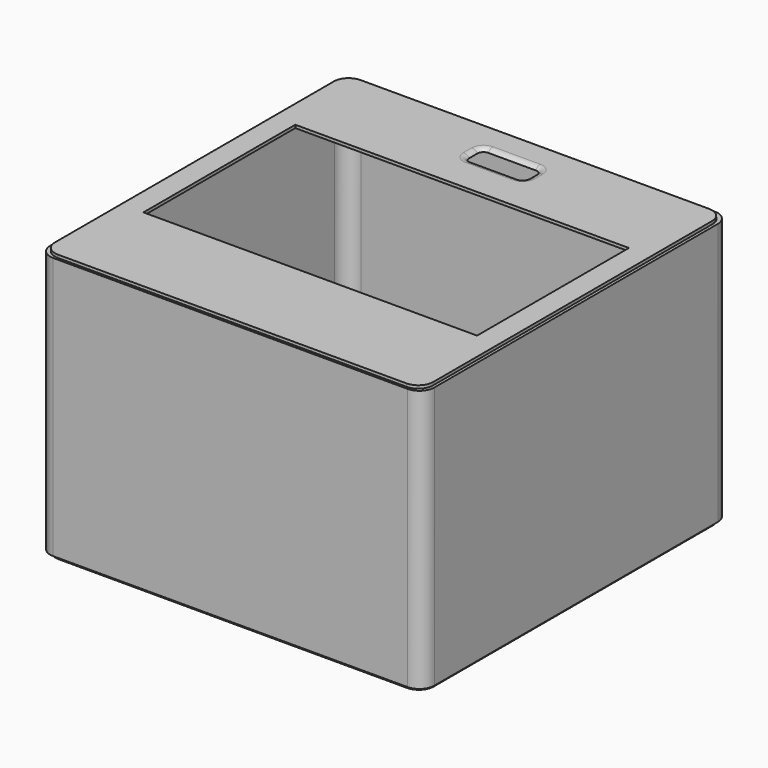
from build123d import *

# Parameters (mm, degrees)
F0_W         = 225
F0_H         = 128
F1_DEPTH     = 2
F2_T1_DEPTH  = 32
F2_T3_DEPTH  = 7
F2_T6_ANGLE  = 90
F2_T8_ANGLE  = 90
F2_T10_ANGLE = 90
F2_T12_ANGLE = 90
F4_DEPTH     = 177
F6_DEPTH     = 2


# Not quite as in the source:
# - a fillet or chamfer that OpenCascade refuses, or shapes differently, is made with other operations: its cross-section is extruded or revolved along the edge and cut away or added


with BuildPart() as f1:
    # F0 (on Top) → F1 (new body)
    with BuildSketch(Plane.XY):
        with BuildLine():
            Line((-120, -130), (115, -130))
            ThreePointArc((115, -130), (122.0710678119, -127.0710678119), (125, -120))
            Line((125, -120), (125, 115))
            ThreePointArc((125, 115), (122.0710678119, 122.0710678119), (115, 125))
            Line((115, 125), (-120, 125))
            ThreePointArc((-120, 125), (-127.0710678119, 122.0710678119), (-130, 115))
            Line((-130, 115), (-130, -120))
            ThreePointArc((-130, -120), (-127.0710678119, -127.0710678119), (-120, -130))
        make_face()
        with Locations((-2.5000095367, -0.2505254149)):
            Rectangle(F0_W, F0_H, mode=Mode.SUBTRACT)
        with BuildLine():
            Line((-18.0000054687, 105.1618295312), (13.9999945313, 105.1618295312))
            ThreePointArc((13.9999945313, 105.1618295312), (16.828421656, 103.9902566559), (17.9999945313, 101.1618295312))
            Line((17.9999945313, 101.1618295312), (17.9999945313, 94.1618295312))
            ThreePointArc((17.9999945313, 94.1618295312), (16.828421656, 91.3334024064), (13.9999945313, 90.1618295312))
            Line((13.9999945313, 90.1618295312), (-18.0000054687, 90.1618295312))
            ThreePointArc((-18.0000054687, 90.1618295312), (-20.8284325935, 91.3334024064), (-22.0000054687, 94.1618295312))
            Line((-22.0000054687, 94.1618295312), (-22.0000054687, 101.1618295312))
            ThreePointArc((-22.0000054687, 101.1618295312), (-20.8284325935, 103.9902566559), (-18.0000054687, 105.1618295312))
        make_face(mode=Mode.SUBTRACT)
    extrude(amount=F1_DEPTH)

    # F2: fillet of radius 5 on 1 edges, made by hand

    # F2_s2 → F2_t1 (cut)
    with BuildSketch(Plane.YZ.offset(-18.0000054687)):
        with BuildLine():
            ThreePointArc((90.1618295312, 0), (88.3978975087, 1.472135955), (86.1618295312, 2))
            Line((86.1618295312, 2), (90.1618295312, 2))
            Line((90.1618295312, 2), (90.1618295312, 0))
        make_face()
        with BuildLine():
            ThreePointArc((105.1618295312, 0), (106.9257615537, 1.472135955), (109.1618295312, 2))
            Line((109.1618295312, 2), (105.1618295312, 2))
            Line((105.1618295312, 2), (105.1618295312, 0))
        make_face()
    extrude(amount=F2_T1_DEPTH, mode=Mode.SUBTRACT)

    # F2_s4 → F2_t3 (cut)
    with BuildSketch(Plane.XZ.offset(-101.1618295312)):
        with BuildLine():
            ThreePointArc((-22.0000054687, 0), (-23.7639374912, 1.472135955), (-26.0000054687, 2))
            Line((-26.0000054687, 2), (-22.0000054687, 2))
            Line((-22.0000054687, 2), (-22.0000054687, 0))
        make_face()
        with BuildLine():
            ThreePointArc((17.9999945313, 0), (19.7639265538, 1.472135955), (21.9999945313, 2))
            Line((21.9999945313, 2), (17.9999945313, 2))
            Line((17.9999945313, 2), (17.9999945313, 0))
        make_face()
    extrude(amount=F2_T3_DEPTH, mode=Mode.SUBTRACT)

    # F2_s5 → F2_t6 (revolve, cut)
    with BuildSketch(Plane.XZ.offset(-94.1618295312)):
        with BuildLine():
            ThreePointArc((17.9999945313, 0), (19.7639265538, 1.472135955), (21.9999945313, 2))
            Line((21.9999945313, 2), (17.9999945313, 2))
            Line((17.9999945313, 2), (17.9999945313, 0))
        make_face()
    revolve(axis=Axis((13.9999945313, 94.1618295312, 2), (0, 0, -1)), revolution_arc=F2_T6_ANGLE, mode=Mode.SUBTRACT)

    # F2_s7 → F2_t8 (revolve, cut)
    with BuildSketch(Plane.YZ.offset(-18.0000054687)):
        with BuildLine():
            ThreePointArc((90.1618295312, 0), (88.3978975087, 1.472135955), (86.1618295312, 2))
            Line((86.1618295312, 2), (90.1618295312, 2))
            Line((90.1618295312, 2), (90.1618295312, 0))
        make_face()
    revolve(axis=Axis((-18.0000054687, 94.1618295312, 2), (0, 0, -1)), revolution_arc=F2_T8_ANGLE, mode=Mode.SUBTRACT)

    # F2_s9 → F2_t10 (revolve, cut)
    with BuildSketch(Plane.XZ.offset(-101.1618295312)):
        with BuildLine():
            ThreePointArc((-22.0000054687, 0), (-23.7639374912, 1.472135955), (-26.0000054687, 2))
            Line((-26.0000054687, 2), (-22.0000054687, 2))
            Line((-22.0000054687, 2), (-22.0000054687, 0))
        make_face()
    revolve(axis=Axis((-18.0000054687, 101.1618295312, 2), (0, 0, -1)), revolution_arc=F2_T10_ANGLE, mode=Mode.SUBTRACT)

    # F2_s11 → F2_t12 (revolve, cut)
    with BuildSketch(Plane.YZ.offset(13.9999945313)):
        with BuildLine():
            ThreePointArc((105.1618295312, 0), (106.9257615537, 1.472135955), (109.1618295312, 2))
            Line((109.1618295312, 2), (105.1618295312, 2))
            Line((105.1618295312, 2), (105.1618295312, 0))
        make_face()
    revolve(axis=Axis((13.9999945313, 101.1618295312, 2), (0, 0, -1)), revolution_arc=F2_T12_ANGLE, mode=Mode.SUBTRACT)


with BuildPart() as f4:
    # F3 (on Top) → F4 (new body)
    with BuildSketch(Plane.XY):
        with BuildLine():
            Line((-121.9999992847, -131.5808296204), (117.0000007153, -131.5808296204))
            ThreePointArc((117.0000007153, -131.5808296204), (124.0710685271, -128.6518974322), (127.0000007153, -121.5808296204))
            Line((127.0000007153, -121.5808296204), (127.0000007153, 117.4191703796))
            ThreePointArc((127.0000007153, 117.4191703796), (124.0710685271, 124.4902381915), (117.0000007153, 127.4191703796))
            Line((117.0000007153, 127.4191703796), (-121.9999992847, 127.4191703796))
            ThreePointArc((-121.9999992847, 127.4191703796), (-129.0710670966, 124.4902381915), (-131.9999992847, 117.4191703796))
            Line((-131.9999992847, 117.4191703796), (-131.9999992847, -121.5808296204))
            ThreePointArc((-131.9999992847, -121.5808296204), (-129.0710670966, -128.6518974322), (-121.9999992847, -131.5808296204))
        make_face()
        with BuildLine():
            ThreePointArc((125.0000007153, -119.5808296204), (122.0710685271, -126.6518974322), (115.0000007153, -129.5808296204))
            Line((115.0000007153, -129.5808296204), (-119.9999992847, -129.5808296204))
            ThreePointArc((-119.9999992847, -129.5808296204), (-127.0710670966, -126.6518974322), (-129.9999992847, -119.5808296204))
            Line((-129.9999992847, -119.5808296204), (-129.9999992847, 115.4191703796))
            ThreePointArc((-129.9999992847, 115.4191703796), (-127.0710670966, 122.4902381915), (-119.9999992847, 125.4191703796))
            Line((-119.9999992847, 125.4191703796), (115.0000007153, 125.4191703796))
            ThreePointArc((115.0000007153, 125.4191703796), (122.0710685271, 122.4902381915), (125.0000007153, 115.4191703796))
            Line((125.0000007153, 115.4191703796), (125.0000007153, -119.5808296204))
        make_face(mode=Mode.SUBTRACT)
    extrude(amount=-F4_DEPTH)


with BuildPart() as f6:
    # F5 (on face) → F6 (new body)
    with BuildSketch(Plane(origin=(0, 0, -177), x_dir=(1, 0, 0), z_dir=(0, 0, -1))):
        with BuildLine():
            Line((-120, -125.4191703796), (115, -125.4191703796))
            ThreePointArc((115, -125.4191703796), (122.0710678119, -122.4902381915), (125, -115.4191703796))
            Line((125, -115.4191703796), (125, 119.5808296204))
            ThreePointArc((125, 119.5808296204), (122.0710678119, 126.6518974322), (115, 129.5808296204))
            Line((115, 129.5808296204), (-120, 129.5808296204))
            ThreePointArc((-120, 129.5808296204), (-127.0710678119, 126.6518974322), (-130, 119.5808296204))
            Line((-130, 119.5808296204), (-130, -115.4191703796))
            ThreePointArc((-130, -115.4191703796), (-127.0710678119, -122.4902381915), (-120, -125.4191703796))
        make_face()
    extrude(amount=F6_DEPTH)


solid = Compound([f1.part, f4.part, f6.part])
